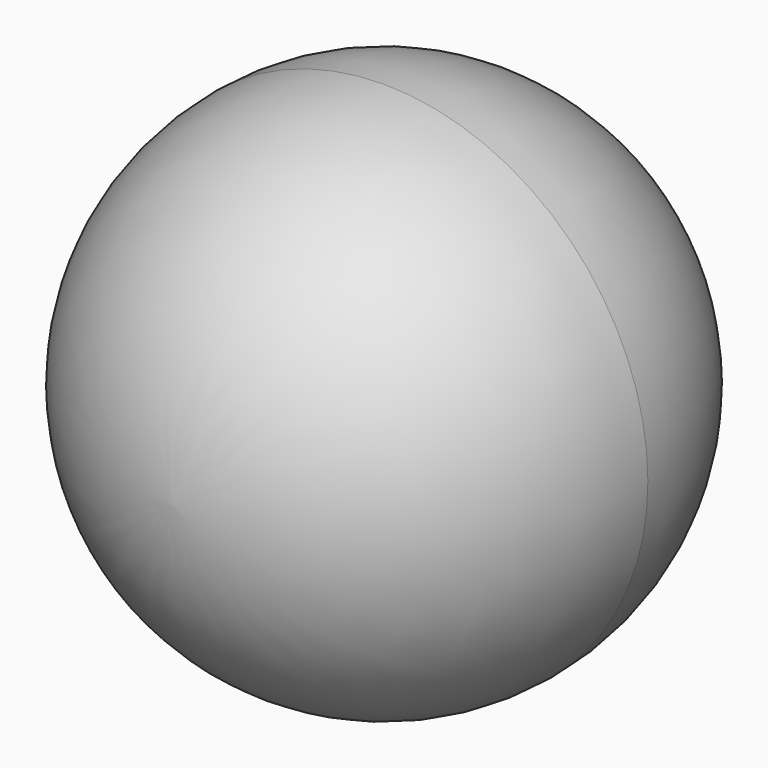
from build123d import *

# Parameters (mm, degrees)
F0_R     = 6.35
F1_DEPTH = 12.7
F2_R     = 6.34999


# Not quite as in the source:
# - a fillet or chamfer is up to 0.001 mm smaller than in the source, because OpenCascade refuses the exact size


with BuildPart() as f1:
    # F0 (on Front) → F1 (new body)
    with BuildSketch(Plane.XZ):
        Circle(F0_R)
    extrude(amount=F1_DEPTH)

    # F2 (radius 6.35 in the source; OpenCascade refuses exactly that, so slightly less here)
    f2_edges = [f1.edges().sort_by_distance(p)[0] for p in [
        (-6.35, -12.7, 0),
        (-6.35, 0, 0),
    ]]
    fillet(f2_edges, radius=F2_R)


solid = f1.part
